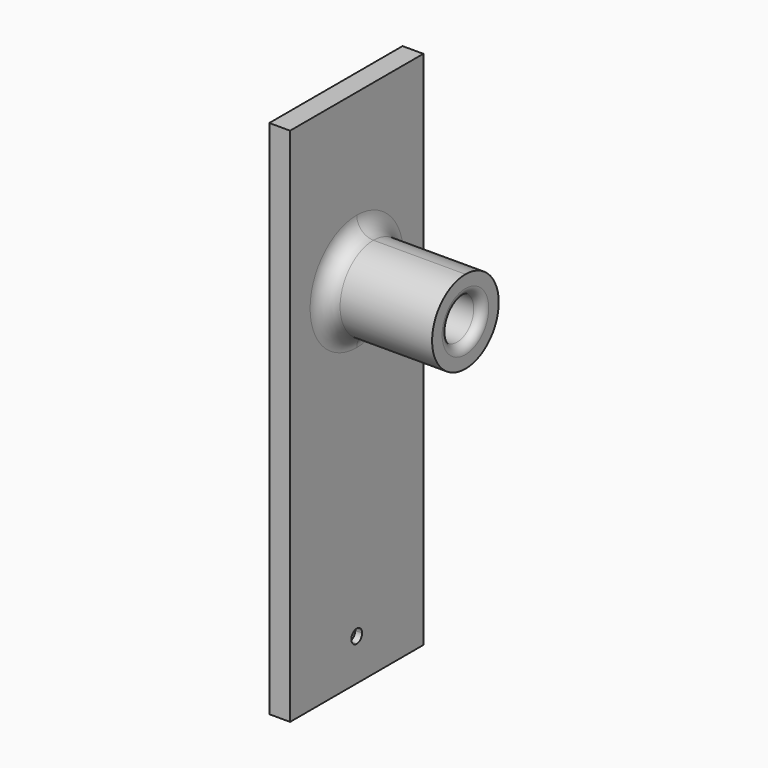
from build123d import *

# Parameters (mm, degrees)
F1_DEPTH = 6.35
F2_DEPTH = 39.497
F3_SIZE2 = 4.2672
F3_SIZE  = 2.7178
F4_R     = 5.08


# Not quite as in the source:
# - a fillet or chamfer that OpenCascade refuses, or shapes differently, is made with other operations: its cross-section is extruded or revolved along the edge and cut away or added


with BuildPart() as f1:
    # F0 (on Right) → F1 (new body)
    with BuildSketch(Plane.YZ):
        with BuildLine():
            Line((0, 79.375), (-25.4, 79.375))
            Line((-25.4, 79.375), (-25.4, -79.375))
            Line((-25.4, -79.375), (0, -79.375))
            Line((0, -79.375), (0, -68.7324))
            ThreePointArc((0, -68.7324), (-2.0574, -66.675), (0, -64.6176))
            Line((0, -64.6176), (0, -53.975))
            Line((0, -53.975), (0, -41.275))
            Line((0, -41.275), (0, 15.875))
            ThreePointArc((0, 15.875), (-12.7, 28.575), (0, 41.275))
            Line((0, 41.275), (0, 79.375))
        make_face()
        with BuildLine():
            Line((25.4, 79.375), (0, 79.375))
            Line((0, 79.375), (0, 41.275))
            ThreePointArc((0, 41.275), (8.9802561211, 37.5552561211), (12.7, 28.575))
            ThreePointArc((12.7, 28.575), (8.9802561211, 19.5947438789), (0, 15.875))
            Line((0, 15.875), (0, -41.275))
            Line((0, -41.275), (0, -53.975))
            Line((0, -53.975), (0, -64.6176))
            ThreePointArc((0, -64.6176), (1.4548014916, -65.2201985084), (2.0574, -66.675))
            ThreePointArc((2.0574, -66.675), (1.4548014916, -68.1298014916), (0, -68.7324))
            Line((0, -68.7324), (0, -79.375))
            Line((0, -79.375), (25.4, -79.375))
            Line((25.4, -79.375), (25.4, 79.375))
        make_face()
        with BuildLine():
            Line((0, 34.925), (0, 41.275))
            ThreePointArc((0, 41.275), (-12.7, 28.575), (0, 15.875))
            Line((0, 15.875), (0, 22.225))
            ThreePointArc((0, 22.225), (-6.35, 28.575), (0, 34.925))
        make_face()
        with BuildLine():
            ThreePointArc((12.7, 28.575), (8.9802561211, 37.5552561211), (0, 41.275))
            Line((0, 41.275), (0, 34.925))
            ThreePointArc((0, 34.925), (4.4901280605, 33.0651280605), (6.35, 28.575))
            ThreePointArc((6.35, 28.575), (4.4901280605, 24.0848719395), (0, 22.225))
            Line((0, 22.225), (0, 15.875))
            ThreePointArc((0, 15.875), (8.9802561211, 19.5947438789), (12.7, 28.575))
        make_face()
    extrude(amount=F1_DEPTH)

    # F0 (on Right) → F2 (join)
    with BuildSketch(Plane.YZ):
        with BuildLine():
            Line((0, 34.925), (0, 41.275))
            ThreePointArc((0, 41.275), (-12.7, 28.575), (0, 15.875))
            Line((0, 15.875), (0, 22.225))
            ThreePointArc((0, 22.225), (-6.35, 28.575), (0, 34.925))
        make_face()
        with BuildLine():
            ThreePointArc((12.7, 28.575), (8.9802561211, 37.5552561211), (0, 41.275))
            Line((0, 41.275), (0, 34.925))
            ThreePointArc((0, 34.925), (4.4901280605, 33.0651280605), (6.35, 28.575))
            ThreePointArc((6.35, 28.575), (4.4901280605, 24.0848719395), (0, 22.225))
            Line((0, 22.225), (0, 15.875))
            ThreePointArc((0, 15.875), (8.9802561211, 19.5947438789), (12.7, 28.575))
        make_face()
    extrude(amount=F2_DEPTH)

    # F3
    f3_edges = [f1.edges().sort_by_distance(p)[0] for p in [
        (0, 0, -68.7324),
    ]]
    f3_side = f1.faces().sort_by_distance((0, 0, -0.344897))[0]
    chamfer(f3_edges, length=F3_SIZE, length2=F3_SIZE2, reference=f3_side)

    # F4
    f4_edges = [f1.edges().sort_by_distance(p)[0] for p in [
        (6.35, 0, 41.275),
    ]]
    fillet(f4_edges, radius=F4_R)

    # F5: fillet of radius 2.54 on 1 edges, made by hand

    # F5_s1 → F5_t2 (revolve, cut)
    with BuildSketch(Plane.XZ):
        with BuildLine():
            ThreePointArc((39.497, 37.465), (38.7530512242, 35.6689487758), (36.957, 34.925))
            Line((36.957, 34.925), (39.497, 34.925))
            Line((39.497, 34.925), (39.497, 37.465))
        make_face()
    revolve(axis=Axis((39.497, 0, 28.575), (-1, 0, 0)), mode=Mode.SUBTRACT)


solid = f1.part
